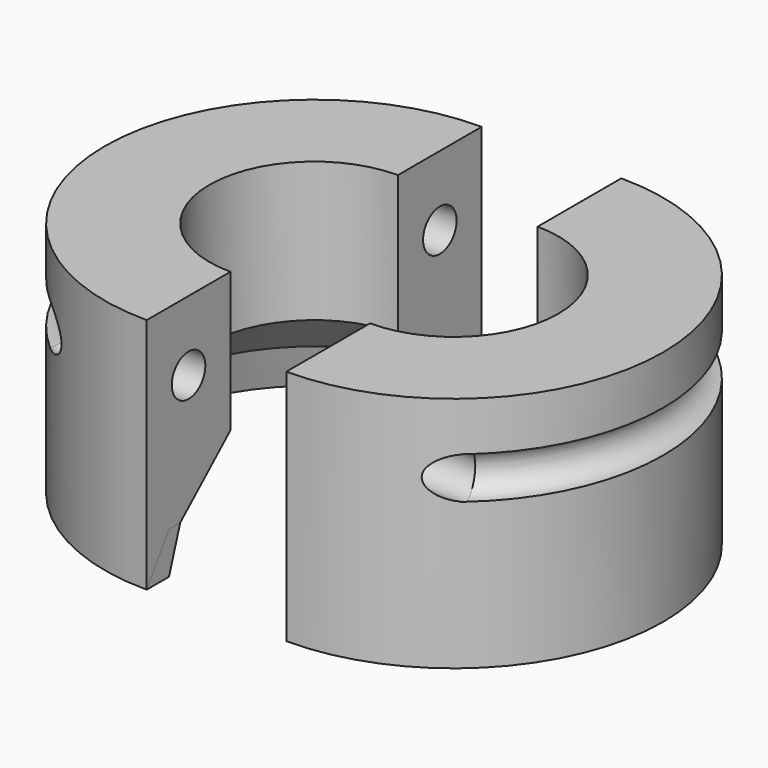
from build123d import *

# Parameters (mm, degrees)
F1_DEPTH       = 10
F3_R           = 1.5
F4_DEPTH       = 25
F5_ANGLE_START = 40
F5_ANGLE       = 100
F7_ANGLE_START = 220
F7_ANGLE       = 100
F8_DEPTH       = 7
F9_DEPTH       = 4


with BuildPart() as f1:
    # F0 (on Top) → F1 (new body)
    with BuildSketch(Plane.XY):
        with BuildLine():
            Line((-10, 12), (-10, 13))
            ThreePointArc((-10, 13), (-23, 0), (-10, -13))
            Line((-10, -13), (-10, -12))
            ThreePointArc((-10, -12), (-22, 0), (-10, 12))
        make_face()
        with BuildLine():
            Line((-10, 7.5), (-10, 12))
            ThreePointArc((-10, 12), (-22, 0), (-10, -12))
            Line((-10, -12), (-10, -7.5))
            ThreePointArc((-10, -7.5), (-17.5, 0), (-10, 7.5))
        make_face()
        with BuildLine():
            Line((-10, 13), (-10, 15))
            ThreePointArc((-10, 15), (-25, 0), (-10, -15))
            Line((-10, -15), (-10, -13))
            ThreePointArc((-10, -13), (-23, 0), (-10, 13))
        make_face()
    extrude(amount=F1_DEPTH)


with BuildPart() as f1b:
    # F0 (on Top) → F1, piece 2 (new body)
    with BuildSketch(Plane.XY):
        with BuildLine():
            ThreePointArc((0, -13), (13, 0), (0, 13))
            Line((0, 13), (0, 12))
            ThreePointArc((0, 12), (12, 0), (0, -12))
            Line((0, -12), (0, -13))
        make_face()
        with BuildLine():
            ThreePointArc((0, -12), (12, 0), (0, 12))
            Line((0, 12), (0, 7.5))
            ThreePointArc((0, 7.5), (7.5, 0), (0, -7.5))
            Line((0, -7.5), (0, -12))
        make_face()
        with BuildLine():
            ThreePointArc((0, -15), (15, 0), (0, 15))
            Line((0, 15), (0, 13))
            ThreePointArc((0, 13), (13, 0), (0, -13))
            Line((0, -13), (0, -15))
        make_face()
    extrude(amount=F1_DEPTH)


with BuildPart() as f4_tool:
    # F3 (on face) → F4 (new body, symmetric)
    with BuildSketch(Plane(origin=(0, 0, 0), x_dir=(0, -1, 0), z_dir=(-1, 0, 0))):
        with Locations((-11.25, 5)):
            Circle(F3_R)
        with Locations((11.25, 5)):
            Circle(F3_R)
    extrude(amount=F4_DEPTH, both=True)


with BuildPart() as f1_1:
    add(f1.part)

    # F4: cut by f4_tool
    add(f4_tool.part, mode=Mode.SUBTRACT)

    # F6 (on face) → F7 (revolve, cut)
    with BuildSketch(Plane.YZ.offset(-10), mode=Mode.PRIVATE) as f7_sk:
        with BuildLine():
            ThreePointArc((-15, 3.5), (-13.9393398282, 3.9393398282), (-13.5, 5))
            ThreePointArc((-13.5, 5), (-13.9393398282, 6.0606601718), (-15, 6.5))
            Line((-15, 6.5), (-15, 3.5))
        make_face()
    revolve(f7_sk.sketch.rotate(Axis((-10, 0, 6.8141282536), (0, 0, 1)), F7_ANGLE_START), axis=Axis((-10, 0, 6.8141282536), (0, 0, 1)), revolution_arc=F7_ANGLE, mode=Mode.SUBTRACT)

    # F0 (on Top) → F8, piece 2 (join)
    with BuildSketch(Plane.XY):
        with BuildLine():
            Line((-10, 13), (-10, 15))
            ThreePointArc((-10, 15), (-25, 0), (-10, -15))
            Line((-10, -15), (-10, -13))
            ThreePointArc((-10, -13), (-23, 0), (-10, 13))
        make_face()
    extrude(amount=-F8_DEPTH)

    # F0 (on Top) → F9, piece 2 (join)
    with BuildSketch(Plane.XY):
        with BuildLine():
            Line((-10, 12), (-10, 13))
            ThreePointArc((-10, 13), (-23, 0), (-10, -13))
            Line((-10, -13), (-10, -12))
            ThreePointArc((-10, -12), (-22, 0), (-10, 12))
        make_face()
    extrude(amount=-F9_DEPTH)

    # F0 (on Top) → F11 section 0
    with BuildSketch(Plane.XY):
        with BuildLine():
            Line((-10, 7.5), (-10, 12))
            ThreePointArc((-10, 12), (-22, 0), (-10, -12))
            Line((-10, -12), (-10, -7.5))
            ThreePointArc((-10, -7.5), (-17.5, 0), (-10, 7.5))
        make_face()
    # F9_face (on face) → F11 section 1
    with BuildSketch(Plane(origin=(7.9619912864, 0, -4), x_dir=(1, 0, 0), z_dir=(0, 0, -1))):
        with BuildLine():
            Line((-17.9619912864, 12), (-17.9619912864, 13))
            ThreePointArc((-17.9619912864, 13), (-30.9619912864, 0), (-17.9619912864, -13))
            Line((-17.9619912864, -13), (-17.9619912864, -12))
            ThreePointArc((-17.9619912864, -12), (-29.9619912864, 0), (-17.9619912864, 12))
        make_face()
    loft()


with BuildPart() as f1b_1:
    add(f1b.part)

    # F4: cut by f4_tool
    add(f4_tool.part, mode=Mode.SUBTRACT)

    # F3 (on face) → F5 (revolve, cut)
    with BuildSketch(Plane(origin=(0, 0, 0), x_dir=(0, -1, 0), z_dir=(-1, 0, 0)), mode=Mode.PRIVATE) as f5_sk:
        with BuildLine():
            Line((15, 3.5), (15, 6.5))
            ThreePointArc((15, 6.5), (13.5, 5), (15, 3.5))
        make_face()
    revolve(f5_sk.sketch.rotate(Axis((0, 0, 4.2424267518), (0, 0, 1)), F5_ANGLE_START), axis=Axis((0, 0, 4.2424267518), (0, 0, 1)), revolution_arc=F5_ANGLE, mode=Mode.SUBTRACT)

    # F0 (on Top) → F8 (join)
    with BuildSketch(Plane.XY):
        with BuildLine():
            ThreePointArc((0, -15), (15, 0), (0, 15))
            Line((0, 15), (0, 13))
            ThreePointArc((0, 13), (13, 0), (0, -13))
            Line((0, -13), (0, -15))
        make_face()
    extrude(amount=-F8_DEPTH)

    # F0 (on Top) → F9 (join)
    with BuildSketch(Plane.XY):
        with BuildLine():
            ThreePointArc((0, -13), (13, 0), (0, 13))
            Line((0, 13), (0, 12))
            ThreePointArc((0, 12), (12, 0), (0, -12))
            Line((0, -12), (0, -13))
        make_face()
    extrude(amount=-F9_DEPTH)

    # F0 (on Top) → F10 section 0
    with BuildSketch(Plane.XY):
        with BuildLine():
            ThreePointArc((0, -12), (12, 0), (0, 12))
            Line((0, 12), (0, 7.5))
            ThreePointArc((0, 7.5), (7.5, 0), (0, -7.5))
            Line((0, -7.5), (0, -12))
        make_face()
    # F9_face (on face) → F10 section 1
    with BuildSketch(Plane(origin=(7.9619912864, 0, -4), x_dir=(1, 0, 0), z_dir=(0, 0, -1))):
        with BuildLine():
            Line((-7.9619912864, -12), (-7.9619912864, -13))
            ThreePointArc((-7.9619912864, -13), (5.0380087136, 0), (-7.9619912864, 13))
            Line((-7.9619912864, 13), (-7.9619912864, 12))
            ThreePointArc((-7.9619912864, 12), (4.0380087136, 0), (-7.9619912864, -12))
        make_face()
    loft()

    # F9_face (on face) → F12 section 0
    with BuildSketch(Plane(origin=(7.9619912864, 0, -4), x_dir=(1, 0, 0), z_dir=(0, 0, -1))):
        with BuildLine():
            Line((-7.9619912864, -12), (-7.9619912864, -13))
            ThreePointArc((-7.9619912864, -13), (5.0380087136, 0), (-7.9619912864, 13))
            Line((-7.9619912864, 13), (-7.9619912864, 12))
            ThreePointArc((-7.9619912864, 12), (4.0380087136, 0), (-7.9619912864, -12))
        make_face()
    # F8_face (on face) → F12 section 1
    with BuildSketch(Plane(origin=(8.9278344268, 0, -7), x_dir=(1, 0, 0), z_dir=(0, 0, -1))):
        with BuildLine():
            Line((-8.9278344268, -13), (-8.9278344268, -15))
            ThreePointArc((-8.9278344268, -15), (6.0721655732, 0), (-8.9278344268, 15))
            Line((-8.9278344268, 15), (-8.9278344268, 13))
            ThreePointArc((-8.9278344268, 13), (4.0721655732, 0), (-8.9278344268, -13))
        make_face()
    loft()


with BuildPart() as f13:
    # F9_face (on face) → F13 section 0
    with BuildSketch(Plane(origin=(7.9619912864, 0, -4), x_dir=(1, 0, 0), z_dir=(0, 0, -1))):
        with BuildLine():
            Line((-17.9619912864, 12), (-17.9619912864, 13))
            ThreePointArc((-17.9619912864, 13), (-30.9619912864, 0), (-17.9619912864, -13))
            Line((-17.9619912864, -13), (-17.9619912864, -12))
            ThreePointArc((-17.9619912864, -12), (-29.9619912864, 0), (-17.9619912864, 12))
        make_face()
    # F8_face (on face) → F13 section 1
    with BuildSketch(Plane(origin=(8.9278344268, 0, -7), x_dir=(1, 0, 0), z_dir=(0, 0, -1))):
        with BuildLine():
            Line((-18.9278344268, 13), (-18.9278344268, 15))
            ThreePointArc((-18.9278344268, 15), (-33.9278344268, 0), (-18.9278344268, -15))
            Line((-18.9278344268, -15), (-18.9278344268, -13))
            ThreePointArc((-18.9278344268, -13), (-31.9278344268, 0), (-18.9278344268, 13))
        make_face()
    loft()


solid = Compound([f1_1.part, f1b_1.part, f13.part])
